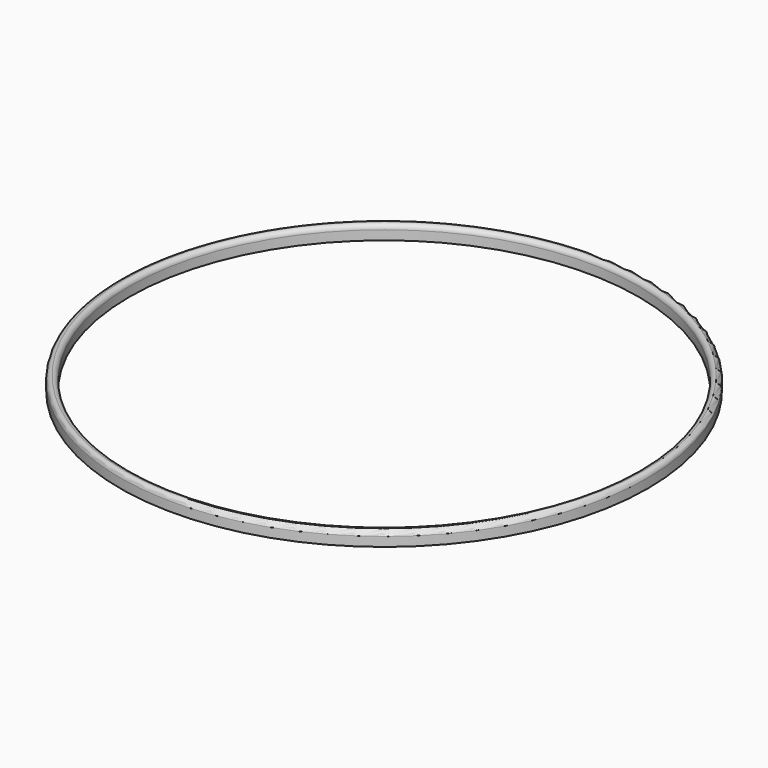
from build123d import *

# Parameters (mm, degrees)
F0_R     = 85
F0_R_2   = 82
F1_DEPTH = 4.5
F2_R     = 1.49999


# Not quite as in the source:
# - a fillet or chamfer is up to 0.001 mm smaller than in the source, because OpenCascade refuses the exact size


with BuildPart() as f1:
    # F0 (on Top) → F1 (new body)
    with BuildSketch(Plane.XY):
        Circle(F0_R)
        Circle(F0_R_2, mode=Mode.SUBTRACT)
    extrude(amount=F1_DEPTH)

    # F2 (radius 1.5 in the source; OpenCascade refuses exactly that, so slightly less here)
    f2_edges = [f1.edges().sort_by_distance(p)[0] for p in [
        (-82, 0, 4.5),
        (-85, 0, 4.5),
    ]]
    fillet(f2_edges, radius=F2_R)


solid = f1.part
